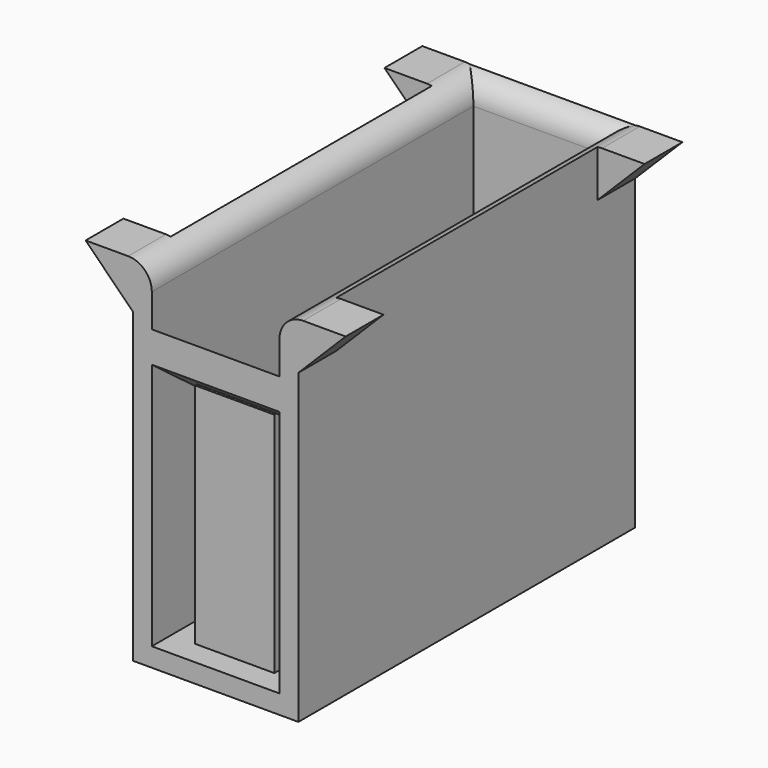
from build123d import *

# Parameters (mm, degrees)
F0_W          = 35
F0_H          = 89
F1_DEPTH      = 63
F2_T          = -4
F3_W          = 27
F3_H          = 7.0524177253
F4_DEPTH      = 4.3
F5_DEPTH      = 5.2
F7_DEPTH      = 12
F9_DEPTH      = 28.5
F8_W          = 16.7951798066
F8_H          = 6.5415552817
F10_DEPTH     = 15.6
F8_W_2        = 16.8639151379
F8_H_2        = 7.3436973616
F11_DEPTH     = 29.2
F8_W_3        = 16.7673844844
F8_H_3        = 8.8219475001
F12_DEPTH     = 48.1
F13_W         = 10
F13_H         = 10
F14_DEPTH     = 10
F15_W         = 10
F15_H         = 10
F16_DEPTH     = 10
F19_DEPTH     = 10
F20_DEPTH     = 10
F21_T1_DEPTH  = 97.5
F21_T3_DEPTH  = 27
F21_T8_DEPTH  = 94
F21_T13_DEPTH = 110
F21_T18_DEPTH = 110
F21_T23_DEPTH = 94
F21_T29_DEPTH = 97.5
F21_T35_DEPTH = 39.5
F21_T44_DEPTH = 39.5
F21_T50_DEPTH = 97.5


# Not quite as in the source:
# - a fillet or chamfer that OpenCascade refuses, or shapes differently, is made with other operations: its cross-section is extruded or revolved along the edge and cut away or added


with BuildPart() as f1:
    # F0 (on Top) → F1 (new body)
    with BuildSketch(Plane.XY):
        Rectangle(F0_W, F0_H)
    extrude(amount=F1_DEPTH)

    # F2
    f2_openings = [f1.faces().sort_by_distance(p)[0] for p in [
        (0, 0, 63),
    ]]
    offset(amount=F2_T, openings=f2_openings)

    # F3 (on face) → F4 (cut)
    with BuildSketch(Plane.XY.offset(4)):
        with Locations((0, 36.9737911373)):
            Rectangle(F3_W, F3_H)
    extrude(amount=-F4_DEPTH, mode=Mode.SUBTRACT)

    # F5 (cut): a face of the model
    f5_faces = [f1.faces().sort_by_distance(p)[0] for p in [
        (0, -40.5, 33.5),
    ]]
    extrude(f5_faces, amount=-F5_DEPTH, mode=Mode.SUBTRACT)

    # F7 (add): a face of the model
    f7_faces = [f1.faces().sort_by_distance(p)[0] for p in [
        (-16.5436527827, 0, 63),
    ]]
    extrude(f7_faces, amount=F7_DEPTH)

    # F6 (on face) → F9 (join)
    with BuildSketch(Plane(origin=(13.5, 0, 0), x_dir=(0, -1, 0), z_dir=(-1, 0, 0))):
        Polygon((44.5, 63), (-33.4475822747, 4), (-24.9599814415, 4), (44.5, 56.4169287682), align=None)
    extrude(amount=F9_DEPTH)

    # F8 (on face) → F10 (join)
    with BuildSketch(Plane.XY.offset(4)):
        with Locations((-0.0789728947, 8.664857829)):
            Rectangle(F8_W, F8_H)
    extrude(amount=F10_DEPTH)

    # F8 (on face) → F11 (join)
    with BuildSketch(Plane.XY.offset(4)):
        with Locations((-0.044605229, -10.0223287009)):
            Rectangle(F8_W_2, F8_H_2)
    extrude(amount=F11_DEPTH)

    # F8 (on face) → F12 (join)
    with BuildSketch(Plane.XY.offset(4)):
        with Locations((-0.0928705558, -34.9372858182)):
            Rectangle(F8_W_3, F8_H_3)
    extrude(amount=F12_DEPTH)

    # F13 (on face) → F14 (join)
    with BuildSketch(Plane.YZ.offset(17.5)):
        with Locations((-39.5, 70)):
            Rectangle(F13_W, F13_H)
        with Locations((39.5, 70)):
            Rectangle(F13_W, F13_H)
    extrude(amount=F14_DEPTH)

    # F15 (on face) → F16 (join)
    with BuildSketch(Plane(origin=(-17.5, 0, 0), x_dir=(0, -1, 0), z_dir=(-1, 0, 0))):
        with Locations((-39.5, 70)):
            Rectangle(F15_W, F15_H)
        with Locations((39.5, 70)):
            Rectangle(F15_W, F15_H)
    extrude(amount=F16_DEPTH)

    # F18 (on face) → F19 (cut)
    with BuildSketch(Plane.XZ.offset(44.5)):
        Polygon((-17.5, 65), (-27.5, 75), (-27.5, 65), align=None)
        Polygon((27.5, 75), (17.5, 65), (27.5, 65), align=None)
    extrude(amount=-F19_DEPTH, mode=Mode.SUBTRACT)

    # F17 (on face) → F20 (cut)
    with BuildSketch(Plane(origin=(0, 44.5, 0), x_dir=(-1, 0, 0), z_dir=(0, 1, 0))):
        Polygon((-17.5, 65), (-27.5, 75), (-27.5, 65), align=None)
        Polygon((27.5, 65), (27.5, 75), (17.5, 65), align=None)
    extrude(amount=-F20_DEPTH, mode=Mode.SUBTRACT)

    # F21: fillet of radius 5 on 7 edges, made by hand

    # F21_s2 → F21_t1 (cut)
    with BuildSketch(Plane.XZ.offset(-40.5)):
        with BuildLine():
            ThreePointArc((-18.5, 75), (-14.9644660941, 73.5355339059), (-13.5, 70))
            Line((-13.5, 70), (-13.5, 75))
            Line((-13.5, 75), (-18.5, 75))
        make_face()
        with BuildLine():
            ThreePointArc((18.5, 75), (14.9644660941, 73.5355339059), (13.5, 70))
            Line((13.5, 70), (13.5, 75))
            Line((13.5, 75), (18.5, 75))
        make_face()
    extrude(amount=F21_T1_DEPTH, mode=Mode.SUBTRACT)

    # F21_s4 → F21_t3 (cut)
    with BuildSketch(Plane.YZ.offset(-13.5)):
        with BuildLine():
            ThreePointArc((45.5, 75), (41.9644660941, 73.5355339059), (40.5, 70))
            Line((40.5, 70), (40.5, 75))
            Line((40.5, 75), (45.5, 75))
        make_face()
    extrude(amount=F21_T3_DEPTH, mode=Mode.SUBTRACT)


with BuildPart() as f21_tool6:
    # F21_s7 → F21_t8 (new body)
    with BuildSketch(Plane.XZ.offset(-47)):
        with BuildLine():
            ThreePointArc((-12.5, 75), (-16.0355339059, 73.5355339059), (-17.5, 70))
            Line((-17.5, 70), (-17.5, 75))
            Line((-17.5, 75), (-12.5, 75))
        make_face()
    extrude(amount=F21_T8_DEPTH)

    split(bisect_by=Plane.YZ.offset(-13.5), keep=Keep.TOP)


with BuildPart() as f1_1:
    add(f1.part)

    # F21_t5: cut F21_tool6
    add(f21_tool6.part, mode=Mode.SUBTRACT)


with BuildPart() as f21_tool11:
    # F21_s12 → F21_t13 (new body)
    with BuildSketch(Plane.XZ.offset(57)):
        with BuildLine():
            ThreePointArc((-18.5, 75), (-14.9644660941, 73.5355339059), (-13.5, 70))
            Line((-13.5, 70), (-13.5, 75))
            Line((-13.5, 75), (-18.5, 75))
        make_face()
    extrude(amount=-F21_T13_DEPTH)

    split(bisect_by=Plane.YZ.offset(-17.5), keep=Keep.BOTTOM)


with BuildPart() as f1_2:
    add(f1_1.part)

    # F21_t10: cut F21_tool11
    add(f21_tool11.part, mode=Mode.SUBTRACT)


with BuildPart() as f21_tool16:
    # F21_s17 → F21_t18 (new body)
    with BuildSketch(Plane.XZ.offset(-53)):
        with BuildLine():
            ThreePointArc((18.5, 75), (14.9644660941, 73.5355339059), (13.5, 70))
            Line((13.5, 70), (13.5, 75))
            Line((13.5, 75), (18.5, 75))
        make_face()
    extrude(amount=F21_T18_DEPTH)

    split(bisect_by=Plane.YZ.offset(17.5), keep=Keep.TOP)


with BuildPart() as f1_3:
    add(f1_2.part)

    # F21_t15: cut F21_tool16
    add(f21_tool16.part, mode=Mode.SUBTRACT)


with BuildPart() as f21_tool21:
    # F21_s22 → F21_t23 (new body)
    with BuildSketch(Plane.XZ.offset(47)):
        with BuildLine():
            ThreePointArc((17.5, 70), (16.0355339059, 73.5355339059), (12.5, 75))
            Line((12.5, 75), (17.5, 75))
            Line((17.5, 75), (17.5, 70))
        make_face()
    extrude(amount=-F21_T23_DEPTH)

    split(bisect_by=Plane.YZ.offset(13.5), keep=Keep.BOTTOM)


with BuildPart() as f1_4:
    add(f1_3.part)

    # F21_t20: cut F21_tool21
    add(f21_tool21.part, mode=Mode.SUBTRACT)


with BuildPart() as f21_tool27:
    # F21_s28 → F21_t29 (new body)
    with BuildSketch(Plane.XZ.offset(44.5)):
        with BuildLine():
            ThreePointArc((-18.5, 75), (-14.9644660941, 73.5355339059), (-13.5, 70))
            Line((-13.5, 70), (-13.5, 75))
            Line((-13.5, 75), (-18.5, 75))
        make_face()
    extrude(amount=-F21_T29_DEPTH)

    split(bisect_by=Plane.YZ.offset(-17.5), keep=Keep.TOP)

    split(bisect_by=Plane.XZ.offset(-44.5), keep=Keep.TOP)

    split(bisect_by=Plane.XZ.offset(-40.5), keep=Keep.BOTTOM)


with BuildPart() as f21_tool33:
    # F21_s34 → F21_t35 (new body)
    with BuildSketch(Plane.YZ.offset(13.5)):
        with BuildLine():
            ThreePointArc((45.5, 75), (41.9644660941, 73.5355339059), (40.5, 70))
            Line((40.5, 70), (40.5, 75))
            Line((40.5, 75), (45.5, 75))
        make_face()
    extrude(amount=-F21_T35_DEPTH)

    split(bisect_by=Plane.YZ.offset(-13.5), keep=Keep.BOTTOM)

    split(bisect_by=Plane.XZ.offset(-44.5), keep=Keep.TOP)

    split(bisect_by=Plane(origin=(23.75, 0, 23.75), x_dir=(0, 1, 0), z_dir=(0.7071067812, 0, 0.7071067812)), keep=Keep.TOP)


with BuildPart() as f21_tool27_1:
    add(f21_tool27.part)

    # F21_t39: intersect F21_tool33
    add(f21_tool33.part, mode=Mode.INTERSECT)


with BuildPart() as f1_5:
    add(f1_4.part)

    # F21_t25: cut F21_tool27
    add(f21_tool27_1.part, mode=Mode.SUBTRACT)


with BuildPart() as f21_tool42:
    # F21_s43 → F21_t44 (new body)
    with BuildSketch(Plane.YZ.offset(26)):
        with BuildLine():
            ThreePointArc((45.5, 75), (41.9644660941, 73.5355339059), (40.5, 70))
            Line((40.5, 70), (40.5, 75))
            Line((40.5, 75), (45.5, 75))
        make_face()
    extrude(amount=-F21_T44_DEPTH)

    split(bisect_by=Plane.YZ.offset(13.5), keep=Keep.TOP)

    split(bisect_by=Plane.XZ.offset(-44.5), keep=Keep.TOP)

    split(bisect_by=Plane(origin=(-23.75, 0, 23.75), x_dir=(0, 1, 0), z_dir=(-0.7071067812, 0, 0.7071067812)), keep=Keep.TOP)


with BuildPart() as f21_tool48:
    # F21_s49 → F21_t50 (new body)
    with BuildSketch(Plane.XZ.offset(-53)):
        with BuildLine():
            ThreePointArc((18.5, 75), (14.9644660941, 73.5355339059), (13.5, 70))
            Line((13.5, 70), (13.5, 75))
            Line((13.5, 75), (18.5, 75))
        make_face()
    extrude(amount=F21_T50_DEPTH)

    split(bisect_by=Plane.YZ.offset(17.5), keep=Keep.BOTTOM)

    split(bisect_by=Plane.XZ.offset(-44.5), keep=Keep.TOP)

    split(bisect_by=Plane.XZ.offset(-40.5), keep=Keep.BOTTOM)


with BuildPart() as f21_tool42_1:
    add(f21_tool42.part)

    # F21_t54: intersect F21_tool48
    add(f21_tool48.part, mode=Mode.INTERSECT)


with BuildPart() as f1_6:
    add(f1_5.part)

    # F21_t40: cut F21_tool42
    add(f21_tool42_1.part, mode=Mode.SUBTRACT)


solid = f1_6.part
